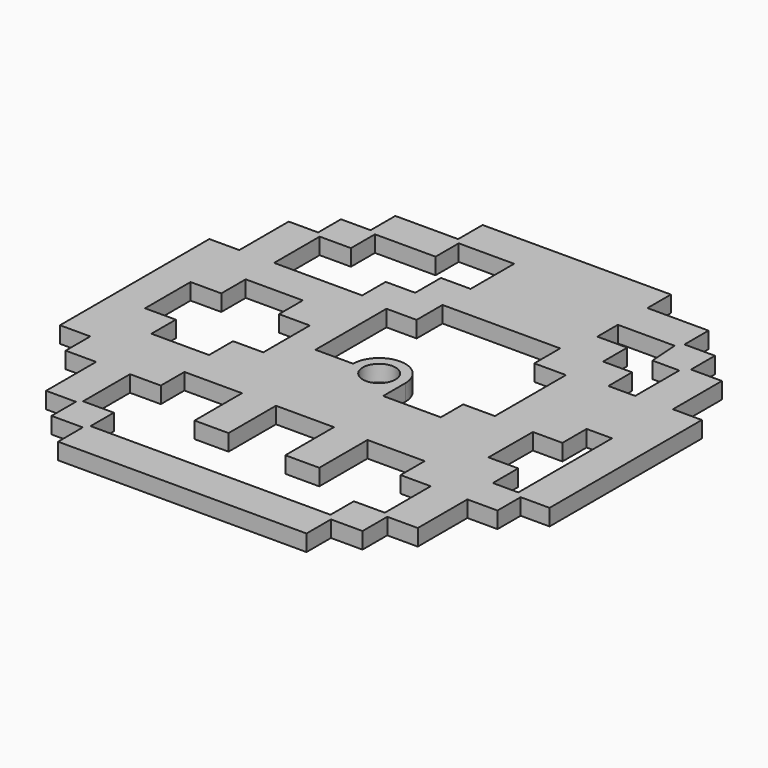
from build123d import *

# Parameters (mm, degrees)
F0_R     = 5
F1_DEPTH = 5


# Not quite as in the source:
# - a feature names something its author has since deleted; it is built from what else it names


with BuildPart() as f1:
    # F0 (on Top) → F1 (new body)
    with BuildSketch(Plane.XY):
        Polygon((28.8361990176, 66.3212267974), (28.8361990176, 75.2581738144), (-28.6278320871, 75.2581738144), (-28.6278320871, 65.9171296439), (-47.7930275365, 65.9171296439), (-47.7930275365, 56.4777807232), (-56.8360119664, 56.4777807232), (-56.8360119664, 47.77079441), (-65.8145548105, 47.77079441), (-65.8145548105, 28.9132569506), (-74.9573593959, 28.9132569506), (-74.9573593959, -28.0682670643), (-65.7083904313, -28.0682670643), (-65.7083904313, -37.4650924841), (-56.4094499535, -37.4650924841), (-56.4094499535, -56.5523879105), (-47.3062752641, -56.5523879105), (-47.3062752641, -65.8493747442), (-37.7622978478, -65.8493747442), (-37.7622978478, -75.2934746653), (38.0699873075, -75.2934746653), (38.0699873075, -65.9706481237), (47.7079034685, -65.9706481237), (47.7079034685, -56.5304698258), (57.015301546, -56.5304698258), (57.015301546, -37.6106819749), (66.2148232459, -37.6106819749), (66.2148232459, -28.7799280069), (75.0426406041, -28.7799280069), (75.0426406041, 29.3137990452), (66.2017579949, 29.3137990452), (66.2017579949, 48.0247353784), (56.7612786638, 48.0247353784), (56.7612786638, 57.1551586931), (47.4673062579, 57.1551586931), (47.4673062579, 66.3212267974), align=None)
        Polygon((19.260561918, -28.5256245699), (36.7241599718, -28.5256245699), (36.7241599718, -37.7505006385), (45.9490339925, -37.7505006385), (45.9490339925, -55.2602632616), (36.4968368924, -55.2602632616), (36.4968368924, -64.1742375536), (-36.7407058072, -64.1742375536), (-36.7407058072, -55.283678321), (-46.1398145742, -55.283678321), (-46.1398145742, -37.3711783135), (-36.7407058072, -37.3711783135), (-36.7407058072, -28.3655547674), (-19.1730977071, -28.3655547674), (-19.1730977071, -46.4431725153), (-8.8080122735, -46.4431725153), (-8.8080122735, -28.3560384318), (8.8979564246, -28.3560384318), (8.8979564246, -46.9153605143), (19.260561918, -46.9153605143), align=None, mode=Mode.SUBTRACT)
        Polygon((56.4795812045, 8.5502099078), (64.2473643763, 8.5502099078), (64.2473643763, -27.2121818547), (56.4795812045, -27.2121818547), (56.4795812045, -17.5323278765), (47.397622189, -17.5323278765), (47.4682605536, -0.6779317695), (56.4795812045, -0.6779317695), align=None, mode=Mode.SUBTRACT)
        Polygon((-37.7697237636, 9.0201110426), (-28.3814624315, 9.0201110426), (-28.3814624315, -8.7280929223), (-37.6123304944, -8.7280929223), (-37.6123304944, -17.8766478564), (-55.2046581313, -17.8766478564), (-55.2046581313, -8.5706945335), (-64.5900750067, -8.5706945335), (-64.5900750067, 8.7840165312), (-55.1995221361, 8.7840165312), (-55.1995221361, 18.0899667823), (-37.7697237636, 18.0899667823), align=None, mode=Mode.SUBTRACT)
        Polygon((-27.1597996025, 64.3126308179), (-10.2554311506, 64.3126308179), (-10.2554311506, 47.7142569757), (-19.3196951095, 47.7142569757), (-19.3196951095, 37.9019094753), (-28.3277433041, 37.9019094753), (-28.3277433041, 28.9398610834), (-55.2046581313, 28.9398610834), (-55.2046581313, 46.3220587686), (-45.6612946386, 46.3220587686), (-45.6612946386, 55.4729318632), (-27.1597996025, 55.4729318632), align=None, mode=Mode.SUBTRACT)
        Polygon((25.6005422263, 27.1866678011), (35.2676995658, 27.1866678011), (35.2676995658, 0.073810573), (25.6005422263, 0.073810573), (25.6005422263, -8.4743950561), (8, -8.4743950561), (-10.3129134285, -8.4743950561), (-10.3129134285, 0.073810573), (-19.5128518648, 0.073810573), (-19.5128518648, 27.1866678011), (-10.3129134285, 27.1866678011), (-10.3129134285, 37.0686502221), (25.6005422263, 37.0686502221), align=None, mode=Mode.SUBTRACT)
        Polygon((28.7232235059, 47.3439866557), (28.7232235059, 55.1743970225), (46.070954491, 55.1743970225), (46.6939048371, 45.9046711012), (54.8776176106, 45.9046711012), (54.8776176106, 29.0882760215), (46.6939048371, 29.0882760215), (46.6939048371, 38.1399474098), (37.8293368529, 38.1399474098), (37.8293368529, 47.3439866557), align=None, mode=Mode.SUBTRACT)
        with BuildLine():
            ThreePointArc((-7.9996594927, 0.073810573), (-0.0369056792, -7.9999148727), (8, 0))
            ThreePointArc((8, 0), (0.0369056792, 7.9999148727), (-7.9996594927, 0.073810573))
        make_face()
        Circle(F0_R, mode=Mode.SUBTRACT)
        with BuildLine():
            Line((-10.3129134285, -8.4743950561), (8, -8.4743950561))
            Line((8, -8.4743950561), (8, 0))
            ThreePointArc((8, 0), (-0.0369056792, -7.9999148727), (-7.9996594927, 0.073810573))
            Line((-7.9996594927, 0.073810573), (-10.3129134285, 0.073810573))
            Line((-10.3129134285, 0.073810573), (-10.3129134285, -8.4743950561))
        make_face()
    extrude(amount=F1_DEPTH)


solid = f1.part
